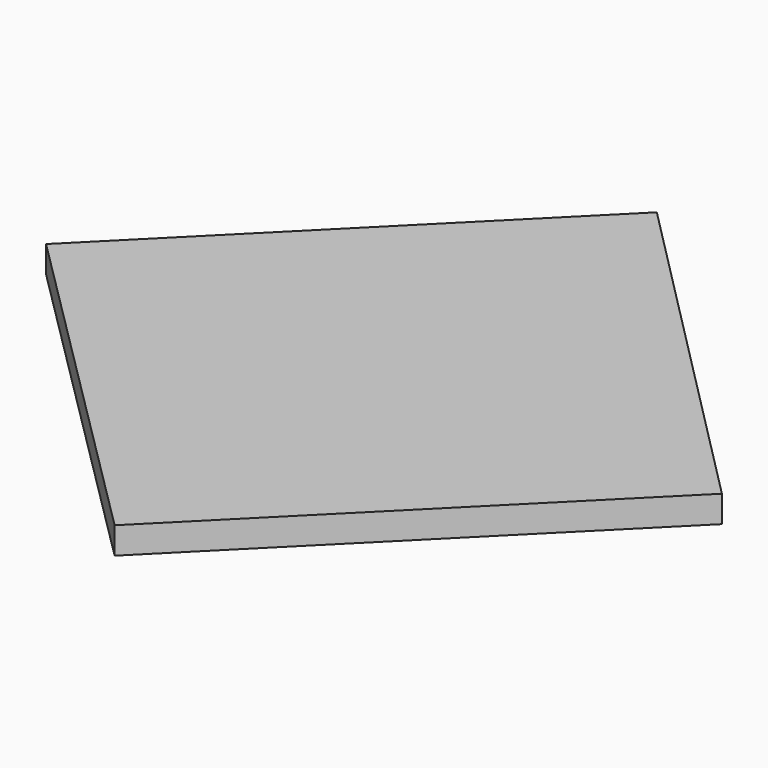
from build123d import *

# Parameters (mm, degrees)
F4_DEPTH = 7.112


# Not quite as in the source:
# - the program builds the solid bodies; features that only make, move or delete a surface that nothing else refers to are left out


with BuildPart() as f4:
    # F2 (on face) → F4 (new body)
    with BuildSketch(Plane.XY):
        Polygon((0, -89.6742220027), (89.421303474, 0), (0, 90.1822071421), (-89.9278558843, 0), align=None)
        Polygon((8.9867543429, -80.634124577), (0, -89.6500274539), (-8.9287396832, -80.634124577), (0, -71.6764245305), align=None, mode=Mode.SUBTRACT)
    extrude(amount=-F4_DEPTH)


with BuildPart() as f4b:
    # F0 (on Top) → F4, piece 2 (new body)
    with BuildSketch(Plane.XY):
        Polygon((89.421303474, 0), (0, 90.1822071421), (-89.9278558843, 0), (0, -89.6742220027), align=None)
    extrude(amount=-F4_DEPTH)


solid = Compound([f4.part, f4b.part])
